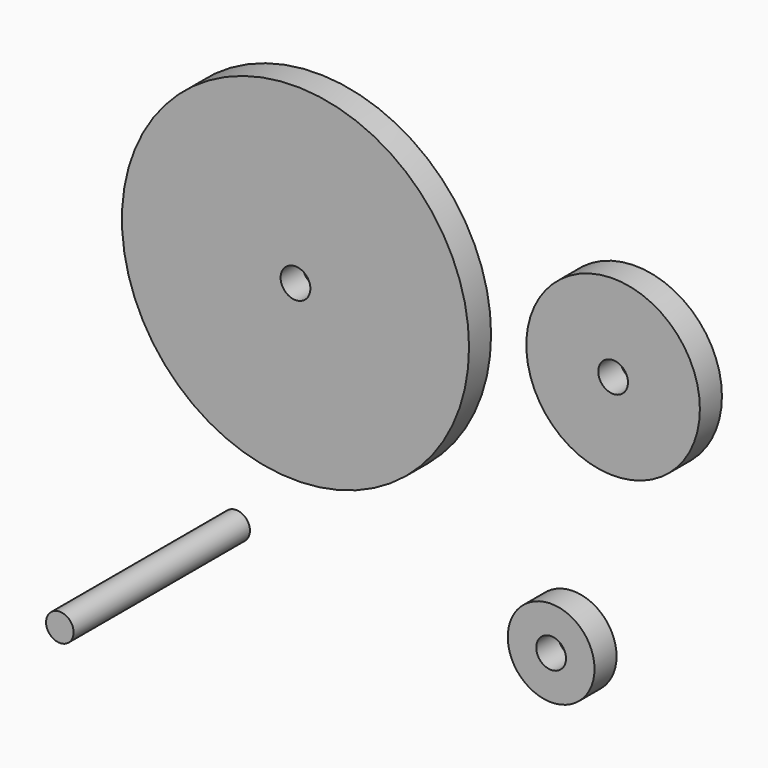
from build123d import *

# Parameters (mm, degrees)
F0_R     = 20
F0_R_2   = 1.7145
F1_DEPTH = 3.175
F2_R     = 10
F2_R_2   = 1.7145
F3_DEPTH = 3.175
F4_R     = 5
F4_R_2   = 1.7145
F5_DEPTH = 3.175
F6_R     = 1.5875
F7_DEPTH = 25.4


# Not quite as in the source:
# - a length typed as a fraction of an inch, garbled in the dataset ("3 / 203.2 mm" for 3/8 in), is restored


with BuildPart() as f1:
    # F0 (on Front) → F1 (new body)
    with BuildSketch(Plane.XZ):
        with Locations((-45.2881418169, 43.5003638268)):
            Circle(F0_R)
        with Locations((-45.2881418169, 43.5003638268)):
            Circle(F0_R_2, mode=Mode.SUBTRACT)
    extrude(amount=F1_DEPTH)


with BuildPart() as f3:
    # F2 (on Front) → F3 (new body)
    with BuildSketch(Plane.XZ):
        with Locations((-8.6867948994, 45.8855852485)):
            Circle(F2_R)
        with Locations((-8.6867948994, 45.8855852485)):
            Circle(F2_R_2, mode=Mode.SUBTRACT)
    extrude(amount=F3_DEPTH)


with BuildPart() as f5:
    # F4 (on Front) → F5 (new body)
    with BuildSketch(Plane.XZ):
        with Locations((-15.8280301839, 15.561719425)):
            Circle(F4_R)
        with Locations((-15.8280301839, 15.561719425)):
            Circle(F4_R_2, mode=Mode.SUBTRACT)
    extrude(amount=F5_DEPTH)


with BuildPart() as f7:
    # F6 (on Front) → F7 (new body)
    with BuildSketch(Plane.XZ):
        with Locations((-54.6649806201, 14.5715419203)):
            Circle(F6_R)
    extrude(amount=F7_DEPTH)


solid = Compound([f1.part, f3.part, f5.part, f7.part])
